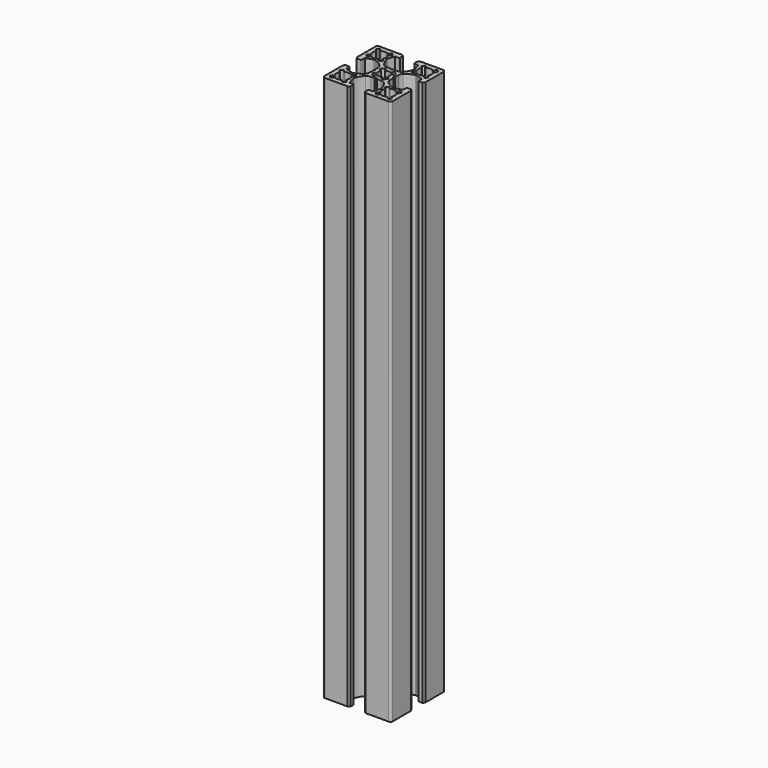
from build123d import *

# Parameters (mm, degrees)
F1_DEPTH = 240


# Not quite as in the source:
# - ends of sketch curves that miss each other by under 0.0002 mm in the source are joined


with BuildPart() as f1:
    # F0 (on Top) → F1 (new body)
    with BuildSketch(Plane.XY):
        with BuildLine():
            Line((-16.817882, -28.053804), (-15.317882, -28.053804))
            ThreePointArc((-15.317882, -28.053804), (-15.2613573135, -27.5251941322), (-15.0943392862, -27.0204878701))
            ThreePointArc((-15.0943392862, -27.0204878701), (-15.1018556445, -26.757114112), (-15.3142900125, -26.6012490693))
            Line((-15.3142900125, -26.6012490693), (-16.055223, -26.467679))
            ThreePointArc((-16.055223, -26.467679), (-16.2747726412, -26.2973161033), (-16.2602657097, -26.0198001716))
            ThreePointArc((-16.2602657097, -26.0198001716), (-15.6451391247, -25.2265468753), (-14.8518861678, -24.611419716))
            ThreePointArc((-14.8518861678, -24.611419716), (-14.574370128, -24.5969122529), (-14.4040070693, -24.8164620125))
            Line((-14.4040070693, -24.8164620125), (-14.270436, -25.557396))
            ThreePointArc((-14.270436, -25.557396), (-14.114570705, -25.7698304515), (-13.8511966819, -25.7773467007))
            ThreePointArc((-13.8511966819, -25.7773467007), (-13.3464912208, -25.6103285465), (-12.817882, -25.553804))
            Line((-12.817882, -25.553804), (-12.817882, -24.053804))
            Line((-12.817882, -24.053804), (-13.317882, -23.553804))
            Line((-13.317882, -23.553804), (-15.035723, -23.553804))
            ThreePointArc((-15.035723, -23.553804), (-15.9762206131, -23.4025693887), (-16.8218943655, -22.9641134932))
            ThreePointArc((-16.8218943655, -22.9641134932), (-18.0925440917, -21.1637239049), (-18.9312372647, -19.1259440756))
            ThreePointArc((-18.9312372647, -19.1259440756), (-18.952848093, -18.864054156), (-18.9054896298, -18.6055767962))
            Line((-18.9054896298, -18.6055767962), (-17.917882, -15.553804))
            Line((-17.917882, -15.553804), (-16.267882, -15.553804))
            ThreePointArc((-16.267882, -15.553804), (-16.0557499656, -15.4659360344), (-15.967882, -15.253804))
            Line((-15.967882, -15.253804), (-15.967882, -13.553804))
            Line((-15.967882, -13.553804), (-16.767882, -13.053804))
            Line((-16.767882, -13.053804), (-26.817882, -13.053804))
            ThreePointArc((-26.817882, -13.053804), (-27.5249887812, -13.3466972188), (-27.817882, -14.053804))
            Line((-27.817882, -14.053804), (-27.817882, -24.103804))
            Line((-27.817882, -24.103804), (-27.317882, -24.903804))
            Line((-27.317882, -24.903804), (-25.617882, -24.903804))
            ThreePointArc((-25.617882, -24.903804), (-25.4057499656, -24.8159360344), (-25.317882, -24.603804))
            Line((-25.317882, -24.603804), (-25.317882, -22.953804))
            Line((-25.317882, -22.953804), (-22.266108, -21.966196))
            ThreePointArc((-22.266108, -21.966196), (-22.0076307271, -21.9188378518), (-21.7457409226, -21.9404486442))
            ThreePointArc((-21.7457409226, -21.9404486442), (-19.7079616374, -22.7791421598), (-17.907572504, -24.049791567))
            ThreePointArc((-17.907572504, -24.049791567), (-17.4691166439, -24.8954652882), (-17.317882, -25.835963))
            Line((-17.317882, -25.835963), (-17.317882, -27.553804))
            Line((-17.317882, -27.553804), (-16.817882, -28.053804))
        make_face()
        with BuildLine():
            ThreePointArc((-20.1318415243, -16.7176952608), (-19.817882, -18.053804), (-20.1318415243, -19.3899127392))
            ThreePointArc((-20.1318415243, -19.3899127392), (-20.1593135799, -19.5718836819), (-20.0753690344, -19.7356560344))
            Line((-20.0753690344, -19.7356560344), (-19.334799, -20.476227))
            ThreePointArc((-19.334799, -20.476227), (-19.2473630595, -20.6722640002), (-19.3132911489, -20.8765408801))
            ThreePointArc((-19.3132911489, -20.8765408801), (-19.6359009875, -21.2357840182), (-19.9951440617, -21.5583939234))
            ThreePointArc((-19.9951440617, -21.5583939234), (-20.1994212978, -21.6243229782), (-20.3954590344, -21.5368870344))
            Line((-20.3954590344, -21.5368870344), (-21.136029, -20.796316))
            ThreePointArc((-21.136029, -20.796316), (-21.2998015274, -20.7123715492), (-21.4817721923, -20.7398436134))
            ThreePointArc((-21.4817721923, -20.7398436134), (-22.8178815523, -21.053804), (-24.153991138, -20.7398442773))
            ThreePointArc((-24.153991138, -20.7398442773), (-24.3359616819, -20.7123714201), (-24.4997340344, -20.7963159656))
            Line((-24.4997340344, -20.7963159656), (-25.240304, -21.536887))
            ThreePointArc((-25.240304, -21.536887), (-25.4363417022, -21.6243229782), (-25.6406189751, -21.5583939691))
            ThreePointArc((-25.6406189751, -21.5583939691), (-25.9998625153, -21.2357845153), (-26.322472412, -20.8765413318))
            ThreePointArc((-26.322472412, -20.8765413318), (-26.3884009573, -20.6722643134), (-26.3009650344, -20.4762269656))
            Line((-26.3009650344, -20.4762269656), (-25.560394, -19.735656))
            ThreePointArc((-25.560394, -19.735656), (-25.4764494201, -19.5718836819), (-25.5039220121, -19.389913006))
            ThreePointArc((-25.5039220121, -19.389913006), (-25.817882, -18.053804), (-25.5039222773, -16.717694862))
            ThreePointArc((-25.5039222773, -16.717694862), (-25.4764494201, -16.5357243181), (-25.5603939656, -16.3719519656))
            Line((-25.5603939656, -16.3719519656), (-26.300965, -15.631381))
            ThreePointArc((-26.300965, -15.631381), (-26.3884009573, -15.4353436866), (-26.3224724576, -15.2310666314))
            ThreePointArc((-26.3224724576, -15.2310666314), (-25.9998625153, -14.8718234847), (-25.6406193318, -14.549213588))
            ThreePointArc((-25.6406193318, -14.549213588), (-25.4363417022, -14.4832850218), (-25.2403039656, -14.5707209656))
            Line((-25.2403039656, -14.5707209656), (-24.499734, -15.311292))
            ThreePointArc((-24.499734, -15.311292), (-24.3359616819, -15.3952365799), (-24.153991006, -15.3677639879))
            ThreePointArc((-24.153991006, -15.3677639879), (-22.8178815523, -15.053804), (-21.4817720604, -15.3677641214))
            ThreePointArc((-21.4817720604, -15.3677641214), (-21.2998015274, -15.3952364508), (-21.1360294656, -15.3112915344))
            Line((-21.1360294656, -15.3112915344), (-20.395459, -14.570721))
            ThreePointArc((-20.395459, -14.570721), (-20.1994212978, -14.4832850218), (-19.9951440249, -14.5492140309))
            ThreePointArc((-19.9951440249, -14.5492140309), (-19.6359009875, -14.8718239818), (-19.3132911946, -15.2310671567))
            ThreePointArc((-19.3132911946, -15.2310671567), (-19.2473630595, -15.4353439998), (-19.3347989656, -15.6313810344))
            Line((-19.3347989656, -15.6313810344), (-20.075369, -16.371952))
            ThreePointArc((-20.075369, -16.371952), (-20.1593135799, -16.5357243181), (-20.1318415243, -16.7176952608))
        make_face(mode=Mode.SUBTRACT)
        with BuildLine():
            Line((-10.317882, -28.053804), (-8.817882, -28.053804))
            Line((-8.817882, -28.053804), (-8.317882, -27.553804))
            Line((-8.317882, -27.553804), (-8.317882, -25.835963))
            ThreePointArc((-8.317882, -25.835963), (-8.1666472628, -24.8954650055), (-7.7281910149, -24.049790989))
            ThreePointArc((-7.7281910149, -24.049790989), (-5.9278016138, -22.7791417483), (-3.8900220756, -21.9404487353))
            ThreePointArc((-3.8900220756, -21.9404487353), (-3.6281322729, -21.9188378518), (-3.3696549943, -21.9661959825))
            Line((-3.3696549943, -21.9661959825), (-0.317882, -22.953804))
            Line((-0.317882, -22.953804), (-0.317882, -24.603804))
            ThreePointArc((-0.317882, -24.603804), (-0.2300140344, -24.8159360344), (-0.017882, -24.903804))
            Line((-0.017882, -24.903804), (1.682118, -24.903804))
            Line((1.682118, -24.903804), (2.182118, -24.103804))
            Line((2.182118, -24.103804), (2.182118, -14.053804))
            ThreePointArc((2.182118, -14.053804), (1.8892247812, -13.3466972188), (1.182118, -13.053804))
            Line((1.182118, -13.053804), (-8.867882, -13.053804))
            Line((-8.867882, -13.053804), (-9.667882, -13.553804))
            Line((-9.667882, -13.553804), (-9.667882, -15.253804))
            ThreePointArc((-9.667882, -15.253804), (-9.5800140344, -15.4659360344), (-9.367882, -15.553804))
            Line((-9.367882, -15.553804), (-7.717882, -15.553804))
            Line((-7.717882, -15.553804), (-6.730274, -18.605577))
            ThreePointArc((-6.730274, -18.605577), (-6.6829159047, -18.8640542036), (-6.7045263914, -19.1259439149))
            ThreePointArc((-6.7045263914, -19.1259439149), (-7.5432189083, -21.1637239049), (-8.8138685119, -22.9641134339))
            ThreePointArc((-8.8138685119, -22.9641134339), (-9.6595430055, -23.4025692628), (-10.600041, -23.553804))
            Line((-10.600041, -23.553804), (-12.317882, -23.553804))
            Line((-12.317882, -23.553804), (-12.817882, -24.053804))
            Line((-12.817882, -24.053804), (-12.817882, -25.553804))
            ThreePointArc((-12.817882, -25.553804), (-12.2892723342, -25.6103286428), (-11.7845662465, -25.777346543))
            ThreePointArc((-11.7845662465, -25.777346543), (-11.521192295, -25.7698304515), (-11.3653270693, -25.5573959875))
            Line((-11.3653270693, -25.5573959875), (-11.231756, -24.816462))
            ThreePointArc((-11.231756, -24.816462), (-11.061392872, -24.5969122529), (-10.7838767336, -24.6114195492))
            ThreePointArc((-10.7838767336, -24.6114195492), (-9.990624391, -25.2265473595), (-9.3754974572, -26.0198002702))
            ThreePointArc((-9.3754974572, -26.0198002702), (-9.3609903588, -26.2973161033), (-9.5805400125, -26.4676789307))
            Line((-9.5805400125, -26.4676789307), (-10.321473, -26.601249))
            ThreePointArc((-10.321473, -26.601249), (-10.5339073555, -26.757114112), (-10.5414238716, -27.0204879417))
            ThreePointArc((-10.5414238716, -27.0204879417), (-10.3744066428, -27.5251943342), (-10.317882, -28.053804))
        make_face()
        with BuildLine():
            ThreePointArc((-5.5627339656, -19.7356560344), (-5.4787894201, -19.5718836819), (-5.5062620121, -19.389913006))
            ThreePointArc((-5.5062620121, -19.389913006), (-5.820221, -18.053804), (-5.5062614757, -16.7176952608))
            ThreePointArc((-5.5062614757, -16.7176952608), (-5.4787894201, -16.5357243181), (-5.5627339656, -16.3719519656))
            Line((-5.5627339656, -16.3719519656), (-6.303305, -15.631381))
            ThreePointArc((-6.303305, -15.631381), (-6.3907399595, -15.4353436467), (-6.3248118511, -15.2310671199))
            ThreePointArc((-6.3248118511, -15.2310671199), (-6.0022020125, -14.8718239818), (-5.6429589383, -14.5492140766))
            ThreePointArc((-5.6429589383, -14.5492140766), (-5.4386817022, -14.4832850218), (-5.2426439656, -14.5707209656))
            Line((-5.2426439656, -14.5707209656), (-4.502074, -15.311292))
            ThreePointArc((-4.502074, -15.311292), (-4.3383016819, -15.3952365799), (-4.156331006, -15.3677639879))
            ThreePointArc((-4.156331006, -15.3677639879), (-2.8202214477, -15.053804), (-1.484111862, -15.3677637227))
            ThreePointArc((-1.484111862, -15.3677637227), (-1.3021413181, -15.3952365799), (-1.1383689656, -15.3112920344))
            Line((-1.1383689656, -15.3112920344), (-0.397799, -14.570721))
            ThreePointArc((-0.397799, -14.570721), (-0.2017612978, -14.4832850218), (0.0025159751, -14.5492140309))
            ThreePointArc((0.0025159751, -14.5492140309), (0.3617595153, -14.8718234847), (0.684369412, -15.2310666682))
            ThreePointArc((0.684369412, -15.2310666682), (0.7502979573, -15.4353436866), (0.6628620344, -15.6313810344))
            Line((0.6628620344, -15.6313810344), (-0.077709, -16.371952))
            ThreePointArc((-0.077709, -16.371952), (-0.1616535799, -16.5357243181), (-0.1341809879, -16.717694994))
            ThreePointArc((-0.1341809879, -16.717694994), (0.179779, -18.053804), (-0.1341807227, -19.389913138))
            ThreePointArc((-0.1341807227, -19.389913138), (-0.1616535799, -19.5718836819), (-0.0777090344, -19.7356560344))
            Line((-0.0777090344, -19.7356560344), (0.662862, -20.476227))
            ThreePointArc((0.662862, -20.476227), (0.7502979573, -20.6722643134), (0.6843694576, -20.8765413686))
            ThreePointArc((0.6843694576, -20.8765413686), (0.3617595153, -21.2357845153), (0.0025163318, -21.558394412))
            ThreePointArc((0.0025163318, -21.558394412), (-0.2017612978, -21.6243229782), (-0.3977990344, -21.5368870344))
            Line((-0.3977990344, -21.5368870344), (-1.138369, -20.796316))
            ThreePointArc((-1.138369, -20.796316), (-1.3021413181, -20.7123714201), (-1.484111994, -20.7398440121))
            ThreePointArc((-1.484111994, -20.7398440121), (-2.8202214477, -21.053804), (-4.1563309396, -20.7398438786))
            ThreePointArc((-4.1563309396, -20.7398438786), (-4.3383016819, -20.7123714201), (-4.5020740344, -20.7963159656))
            Line((-4.5020740344, -20.7963159656), (-5.242644, -21.536887))
            ThreePointArc((-5.242644, -21.536887), (-5.4386817022, -21.6243229782), (-5.6429589751, -21.5583939691))
            ThreePointArc((-5.6429589751, -21.5583939691), (-6.0022020125, -21.2357840182), (-6.3248118054, -20.8765408433))
            ThreePointArc((-6.3248118054, -20.8765408433), (-6.3907399595, -20.6722643533), (-6.3033045344, -20.4762274656))
            Line((-6.3033045344, -20.4762274656), (-5.5627339656, -19.7356560344))
        make_face(mode=Mode.SUBTRACT)
        with BuildLine():
            Line((-8.317882, -28.553804), (-8.817882, -28.053804))
            Line((-8.817882, -28.053804), (-10.317882, -28.053804))
            ThreePointArc((-10.317882, -28.053804), (-10.3744066428, -28.5824136658), (-10.541424543, -29.0871197535))
            ThreePointArc((-10.541424543, -29.0871197535), (-10.5339073967, -29.3504938095), (-10.3214731621, -29.5063588992))
            Line((-10.3214731621, -29.5063588992), (-9.58054, -29.639929))
            ThreePointArc((-9.58054, -29.639929), (-9.3609903588, -29.8102918967), (-9.3754972903, -30.0878078284))
            ThreePointArc((-9.3754972903, -30.0878078284), (-9.990624391, -30.8810606405), (-10.783877091, -31.496187846))
            ThreePointArc((-10.783877091, -31.496187846), (-11.061392872, -31.5106957471), (-11.2317559307, -31.2911459875))
            Line((-11.2317559307, -31.2911459875), (-11.365327, -30.550212))
            ThreePointArc((-11.365327, -30.550212), (-11.521192112, -30.3377776445), (-11.7845659417, -30.3302611284))
            ThreePointArc((-11.7845659417, -30.3302611284), (-12.2892721322, -30.4972793135), (-12.817882, -30.553804))
            Line((-12.817882, -30.553804), (-12.817882, -32.053804))
            Line((-12.817882, -32.053804), (-12.317882, -32.553804))
            Line((-12.317882, -32.553804), (-10.600041, -32.553804))
            ThreePointArc((-10.600041, -32.553804), (-9.6595430055, -32.7050387372), (-8.813868989, -33.1434949851))
            ThreePointArc((-8.813868989, -33.1434949851), (-7.5432189083, -34.9438840951), (-6.7045257353, -36.9816639244))
            ThreePointArc((-6.7045257353, -36.9816639244), (-6.6829158812, -37.2435533212), (-6.7302739825, -37.5020300057))
            Line((-6.7302739825, -37.5020300057), (-7.717882, -40.553804))
            Line((-7.717882, -40.553804), (-9.367882, -40.553804))
            ThreePointArc((-9.367882, -40.553804), (-9.5800140344, -40.6416719656), (-9.667882, -40.853804))
            Line((-9.667882, -40.853804), (-9.667882, -42.553804))
            Line((-9.667882, -42.553804), (-8.867882, -43.053804))
            Line((-8.867882, -43.053804), (1.182118, -43.053804))
            ThreePointArc((1.182118, -43.053804), (1.8892247812, -42.7609107812), (2.182118, -42.053804))
            Line((2.182118, -42.053804), (2.182118, -32.003804))
            Line((2.182118, -32.003804), (1.682118, -31.203804))
            Line((1.682118, -31.203804), (-0.017882, -31.203804))
            ThreePointArc((-0.017882, -31.203804), (-0.2300140344, -31.2916719656), (-0.317882, -31.503804))
            Line((-0.317882, -31.503804), (-0.317882, -33.153804))
            Line((-0.317882, -33.153804), (-3.369655, -34.141412))
            ThreePointArc((-3.369655, -34.141412), (-3.6281322729, -34.1887701482), (-3.8900220774, -34.1671593558))
            ThreePointArc((-3.8900220774, -34.1671593558), (-5.9278016138, -33.3284662517), (-7.7281909374, -32.0578169295))
            ThreePointArc((-7.7281909374, -32.0578169295), (-8.1666472628, -31.2121429945), (-8.317882, -30.271645))
            Line((-8.317882, -30.271645), (-8.317882, -28.553804))
        make_face()
        with BuildLine():
            ThreePointArc((-5.507146239, -39.3904841188), (-5.8210019909, -38.0543501064), (-5.5069379006, -36.7182650494))
            ThreePointArc((-5.5069379006, -36.7182650494), (-5.4794506299, -36.5362965287), (-5.5633824662, -36.3725174663))
            Line((-5.5633824662, -36.3725174663), (-6.303896, -35.631889))
            ThreePointArc((-6.303896, -35.631889), (-6.3913162338, -35.4358449105), (-6.3253716664, -35.2315732687))
            ThreePointArc((-6.3253716664, -35.2315732687), (-6.0027340882, -34.8723550769), (-5.6434657786, -34.5497732749))
            ThreePointArc((-5.6434657786, -34.5497732749), (-5.4391833549, -34.483860277), (-5.2431524662, -34.5713114663))
            Line((-5.2431524662, -34.5713114663), (-4.50264, -35.31194))
            ThreePointArc((-4.50264, -35.31194), (-4.3388740212, -35.3958977668), (-4.1569008286, -35.3684393446))
            ThreePointArc((-4.1569008286, -35.3684393446), (-2.8207674361, -35.0545840092), (-1.4846830494, -35.3686480994))
            ThreePointArc((-1.4846830494, -35.3686480994), (-1.3027146578, -35.3961343911), (-1.1389359663, -35.3122030337))
            Line((-1.1389359663, -35.3122030337), (-0.398307, -34.57169))
            ThreePointArc((-0.398307, -34.57169), (-0.2022626922, -34.4842688081), (0.0020096134, -34.5502132386))
            ThreePointArc((0.0020096134, -34.5502132386), (0.3612269231, -34.8728519118), (0.6838087251, -35.2321202214))
            ThreePointArc((0.6838087251, -35.2321202214), (0.7497216831, -35.4364023869), (0.6622700337, -35.6324330337))
            Line((0.6622700337, -35.6324330337), (-0.078358, -36.372946))
            ThreePointArc((-0.078358, -36.372946), (-0.1623158238, -36.5367113277), (-0.1348573446, -36.7186841714))
            ThreePointArc((-0.1348573446, -36.7186841714), (0.1789979909, -38.0548178935), (-0.1350659009, -39.3909025518))
            ThreePointArc((-0.1350659009, -39.3909025518), (-0.162552241, -39.5728712621), (-0.0786200338, -39.7366500338))
            Line((-0.0786200338, -39.7366500338), (0.661893, -40.477278))
            ThreePointArc((0.661893, -40.477278), (0.7493132149, -40.6733227364), (0.6833686664, -40.8775947313))
            ThreePointArc((0.6833686664, -40.8775947313), (0.3607308072, -41.2368122042), (0.0014628737, -41.5593938432))
            ThreePointArc((0.0014628737, -41.5593938432), (-0.202819292, -41.625306742), (-0.3988500338, -41.5378560338))
            Line((-0.3988500338, -41.5378560338), (-1.139363, -40.797227))
            ThreePointArc((-1.139363, -40.797227), (-1.303129108, -40.7132702121), (-1.4851017727, -40.7407284571))
            ThreePointArc((-1.4851017727, -40.7407284571), (-2.8212354459, -41.0545839909), (-4.157320149, -40.7405202994))
            ThreePointArc((-4.157320149, -40.7405202994), (-4.3392886912, -40.7130336658), (-4.5030675338, -40.7969654663))
            Line((-4.5030675338, -40.7969654663), (-5.243696, -41.537478))
            ThreePointArc((-5.243696, -41.537478), (-5.4397403476, -41.624898194), (-5.6440121248, -41.5589541549))
            ThreePointArc((-5.6440121248, -41.5589541549), (-6.0032304261, -41.2363165853), (-6.3258123317, -40.8770482671))
            ThreePointArc((-6.3258123317, -40.8770482671), (-6.3917246831, -40.6727656131), (-6.3042730337, -40.4767349663))
            Line((-6.3042730337, -40.4767349663), (-5.563645, -39.736222))
            ThreePointArc((-5.563645, -39.736222), (-5.4796873054, -39.5724564631), (-5.507146239, -39.3904841188))
        make_face(mode=Mode.SUBTRACT)
        with BuildLine():
            ThreePointArc((-15.0943392862, -29.0871201299), (-15.2613573135, -28.5824138678), (-15.317882, -28.053804))
            Line((-15.317882, -28.053804), (-16.817882, -28.053804))
            Line((-16.817882, -28.053804), (-17.317882, -28.553804))
            Line((-17.317882, -28.553804), (-17.317882, -30.271645))
            ThreePointArc((-17.317882, -30.271645), (-17.4691166439, -31.2121427118), (-17.9075726307, -32.0578165326))
            ThreePointArc((-17.9075726307, -32.0578165326), (-19.7079616374, -33.3284658402), (-21.7457409999, -34.1671590005))
            ThreePointArc((-21.7457409999, -34.1671590005), (-22.0076307271, -34.1887701482), (-22.2661080057, -34.1414120175))
            Line((-22.2661080057, -34.1414120175), (-25.317882, -33.153804))
            Line((-25.317882, -33.153804), (-25.317882, -31.503804))
            ThreePointArc((-25.317882, -31.503804), (-25.4057499656, -31.2916719656), (-25.617882, -31.203804))
            Line((-25.617882, -31.203804), (-27.317882, -31.203804))
            Line((-27.317882, -31.203804), (-27.817882, -32.003804))
            Line((-27.817882, -32.003804), (-27.817882, -42.053804))
            ThreePointArc((-27.817882, -42.053804), (-27.5249887812, -42.7609107812), (-26.817882, -43.053804))
            Line((-26.817882, -43.053804), (-16.767882, -43.053804))
            Line((-16.767882, -43.053804), (-15.967882, -42.553804))
            Line((-15.967882, -42.553804), (-15.967882, -40.853804))
            ThreePointArc((-15.967882, -40.853804), (-16.0557499656, -40.6416719656), (-16.267882, -40.553804))
            Line((-16.267882, -40.553804), (-17.917882, -40.553804))
            Line((-17.917882, -40.553804), (-18.905489, -37.50203))
            ThreePointArc((-18.905489, -37.50203), (-18.9528481165, -37.2435533689), (-18.9312375634, -36.9816638775))
            ThreePointArc((-18.9312375634, -36.9816638775), (-18.0925440917, -34.9438840951), (-16.8218944881, -33.1434945661))
            ThreePointArc((-16.8218944881, -33.1434945661), (-15.9762206131, -32.7050386113), (-15.035723, -32.553804))
            Line((-15.035723, -32.553804), (-13.317882, -32.553804))
            Line((-13.317882, -32.553804), (-12.817882, -32.053804))
            Line((-12.817882, -32.053804), (-12.817882, -30.553804))
            ThreePointArc((-12.817882, -30.553804), (-13.3464914228, -30.4972794098), (-13.8511973007, -30.3302616625))
            ThreePointArc((-13.8511973007, -30.3302616625), (-14.114570888, -30.3377776445), (-14.2704359307, -30.5502120125))
            Line((-14.2704359307, -30.5502120125), (-14.404007, -31.291146))
            ThreePointArc((-14.404007, -31.291146), (-14.574370128, -31.5106957471), (-14.8518862664, -31.4961884508))
            ThreePointArc((-14.8518862664, -31.4961884508), (-15.6451391247, -30.8810611247), (-16.260266284, -30.0878081678))
            ThreePointArc((-16.260266284, -30.0878081678), (-16.2747726412, -29.8102918967), (-16.0552229875, -29.6399290693))
            Line((-16.0552229875, -29.6399290693), (-15.31429, -29.506358))
            ThreePointArc((-15.31429, -29.506358), (-15.1018556033, -29.3504938095), (-15.0943392862, -29.0871201299))
        make_face()
        with BuildLine():
            ThreePointArc((-20.0747205338, -36.3725174663), (-20.1586523342, -36.5362963089), (-20.1311656295, -36.7182648157))
            ThreePointArc((-20.1311656295, -36.7182648157), (-19.8171020091, -38.0543498837), (-20.1309575628, -39.3904837201))
            ThreePointArc((-20.1309575628, -39.3904837201), (-20.1584156946, -39.5724564631), (-20.0744580337, -39.7362220337))
            Line((-20.0744580337, -39.7362220337), (-19.33383, -40.476735))
            ThreePointArc((-19.33383, -40.476735), (-19.2463783169, -40.6727656131), (-19.3122908476, -40.8770481227))
            ThreePointArc((-19.3122908476, -40.8770481227), (-19.6348730769, -41.2363160882), (-19.9940910142, -41.5589539824))
            ThreePointArc((-19.9940910142, -41.5589539824), (-20.1983629105, -41.6248982338), (-20.3944070337, -41.5374780337))
            Line((-20.3944070337, -41.5374780337), (-21.135036, -40.796965))
            ThreePointArc((-21.135036, -40.796965), (-21.2988146578, -40.7130336089), (-21.4807828157, -40.7405203705))
            ThreePointArc((-21.4807828157, -40.7405203705), (-22.8168676587, -41.0545839908), (-24.1530013171, -40.7407286377))
            ThreePointArc((-24.1530013171, -40.7407286377), (-24.334973892, -40.7132702121), (-24.4987395337, -40.7972274662))
            Line((-24.4987395337, -40.7972274662), (-25.239253, -41.537856))
            ThreePointArc((-25.239253, -41.537856), (-25.435283708, -41.625306742), (-25.6395657293, -41.5593936639))
            ThreePointArc((-25.6395657293, -41.5593936639), (-25.99883431, -41.2368127014), (-26.3214719824, -40.8775949858))
            ThreePointArc((-26.3214719824, -40.8775949858), (-26.3874162149, -40.6733227364), (-26.2999955337, -40.4772784662))
            Line((-26.2999955337, -40.4772784662), (-25.559483, -39.73665))
            ThreePointArc((-25.559483, -39.73665), (-25.475550759, -39.5728712621), (-25.5030371701, -39.3909025871))
            ThreePointArc((-25.5030371701, -39.3909025871), (-25.8171019909, -38.0548178936), (-25.503246239, -36.7186838812))
            ThreePointArc((-25.503246239, -36.7186838812), (-25.4757871762, -36.5367113277), (-25.5597444663, -36.3729454662))
            Line((-25.5597444663, -36.3729454662), (-26.300374, -35.632433))
            ThreePointArc((-26.300374, -35.632433), (-26.3878247021, -35.4364020339), (-26.3219121524, -35.2321198773))
            ThreePointArc((-26.3219121524, -35.2321198773), (-25.9993304261, -34.8728514147), (-25.6401123794, -34.550213529))
            ThreePointArc((-25.6401123794, -34.550213529), (-25.4358403078, -34.4842688081), (-25.2397959662, -34.5716899662))
            Line((-25.2397959662, -34.5716899662), (-24.499168, -35.312203))
            ThreePointArc((-24.499168, -35.312203), (-24.3353886912, -35.3961343342), (-24.1534201843, -35.3686476295))
            ThreePointArc((-24.1534201843, -35.3686476295), (-22.8173356686, -35.0545840091), (-21.4812022799, -35.3684395628))
            ThreePointArc((-21.4812022799, -35.3684395628), (-21.2992289788, -35.3958977668), (-21.1354629663, -35.3119400337))
            Line((-21.1354629663, -35.3119400337), (-20.39495, -34.571312))
            ThreePointArc((-20.39495, -34.571312), (-20.1989200339, -34.4838602979), (-19.9946378773, -34.5497728476))
            ThreePointArc((-19.9946378773, -34.5497728476), (-19.63536969, -34.8723552987), (-19.312731624, -35.2315735027))
            ThreePointArc((-19.312731624, -35.2315735027), (-19.2467867662, -35.4358449105), (-19.3342069663, -35.6318890337))
            Line((-19.3342069663, -35.6318890337), (-20.0747205338, -36.3725174663))
        make_face(mode=Mode.SUBTRACT)
    extrude(amount=F1_DEPTH)


solid = f1.part
